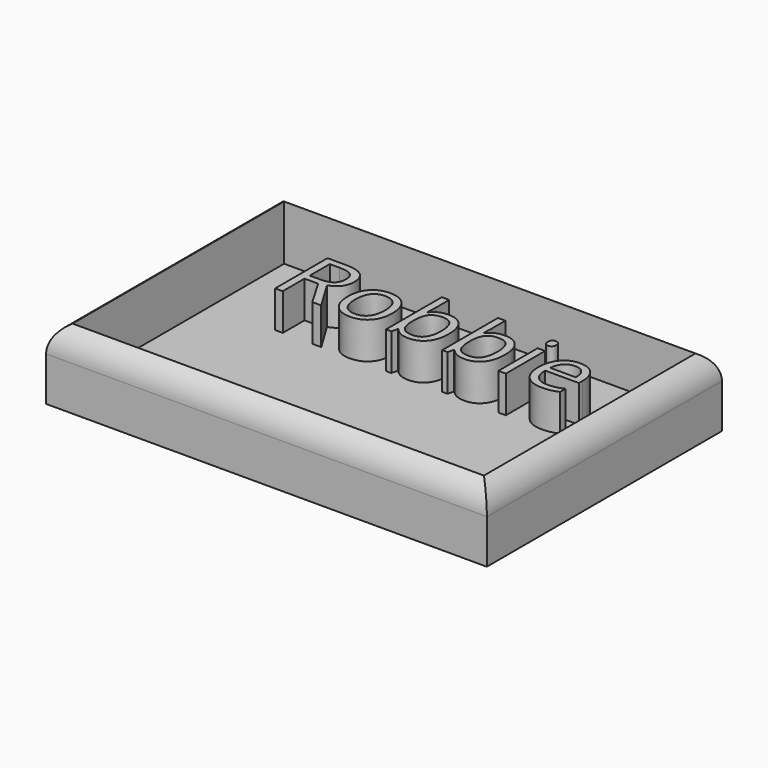
from build123d import *

# Parameters (mm, degrees)
F0_W         = 76.2
F0_H         = 50.8
F1_DEPTH     = 12.7
F2_T         = -2.54
F3_TEXT_SIZE = 15.8467032533
F4_DEPTH     = 6.35
F5_T1_DEPTH  = 101.6
F5_T3_DEPTH  = 76.2


# Not quite as in the source:
# - a fillet or chamfer that OpenCascade refuses, or shapes differently, is made with other operations: its cross-section is extruded or revolved along the edge and cut away or added
# - Text() gives the source's letters only with a copy of the font that has no kerning and outlines rounded to 1/6400 em; it was checked with that copy


with BuildPart() as f1:
    # F0 (on Top) → F1 (new body)
    with BuildSketch(Plane.XY):
        with Locations((3.8507487625, 0.0280697902)):
            Rectangle(F0_W, F0_H)
    extrude(amount=F1_DEPTH)

    # F2
    f2_openings = [f1.faces().sort_by_distance(p)[0] for p in [
        (3.850749, 0.02807, 12.7),
    ]]
    offset(amount=F2_T, openings=f2_openings)

    # F3 (on face) → F4 (join)
    with BuildSketch(Plane.XY.offset(2.54)):
        with Locations((-22.0912002024, 6.9883959368)):
            Text('Robbie', F3_TEXT_SIZE, font='Open Sans', text_align=(TextAlign.LEFT, TextAlign.BOTTOM))
    extrude(amount=F4_DEPTH)

    # F5: fillet of radius 5.08 on 4 edges, made by hand

    # F5_s2 → F5_t1 (cut)
    with BuildSketch(Plane.YZ.offset(-46.9492512375)):
        with BuildLine():
            ThreePointArc((25.4280697902, 7.62), (23.9401722386, 11.2121024484), (20.3480697902, 12.7))
            Line((20.3480697902, 12.7), (25.4280697902, 12.7))
            Line((25.4280697902, 12.7), (25.4280697902, 7.62))
        make_face()
        with BuildLine():
            ThreePointArc((-20.2919302098, 12.7), (-23.8840326582, 11.2121024484), (-25.3719302098, 7.62))
            Line((-25.3719302098, 7.62), (-25.3719302098, 12.7))
            Line((-25.3719302098, 12.7), (-20.2919302098, 12.7))
        make_face()
    extrude(amount=F5_T1_DEPTH, mode=Mode.SUBTRACT)

    # F5_s4 → F5_t3 (cut)
    with BuildSketch(Plane.XZ.offset(-38.1280697902)):
        with BuildLine():
            ThreePointArc((41.9507487625, 7.62), (40.4628512109, 11.2121024484), (36.8707487625, 12.7))
            Line((36.8707487625, 12.7), (41.9507487625, 12.7))
            Line((41.9507487625, 12.7), (41.9507487625, 7.62))
        make_face()
        with BuildLine():
            ThreePointArc((-34.2492512375, 7.62), (-32.7613536859, 11.2121024484), (-29.1692512375, 12.7))
            Line((-29.1692512375, 12.7), (-34.2492512375, 12.7))
            Line((-34.2492512375, 12.7), (-34.2492512375, 7.62))
        make_face()
    extrude(amount=F5_T3_DEPTH, mode=Mode.SUBTRACT)


solid = f1.part
